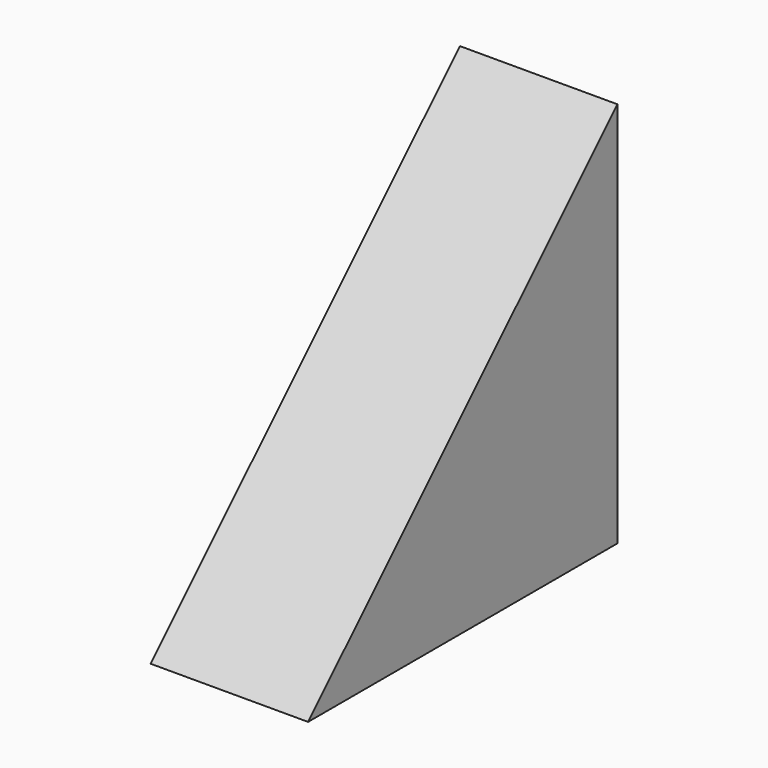
from build123d import *

# Parameters (mm, degrees)
F0_W     = 54
F0_H     = 54
F1_DEPTH = 22
F2_SIZE  = 53.99999


# Not quite as in the source:
# - a fillet or chamfer is up to 0.001 mm smaller than in the source, because OpenCascade refuses the exact size


with BuildPart() as f1:
    # F0 (on Right) → F1 (new body)
    with BuildSketch(Plane.YZ):
        with Locations((16.3859415352, -5.9913944006)):
            Rectangle(F0_W, F0_H)
    extrude(amount=F1_DEPTH)

    # F2 (size 54 in the source; OpenCascade refuses exactly that, so slightly less here)
    f2_edges = [f1.edges().sort_by_distance(p)[0] for p in [
        (11, -10.614058, 21.008606),
    ]]
    chamfer(f2_edges, length=F2_SIZE)


solid = f1.part
